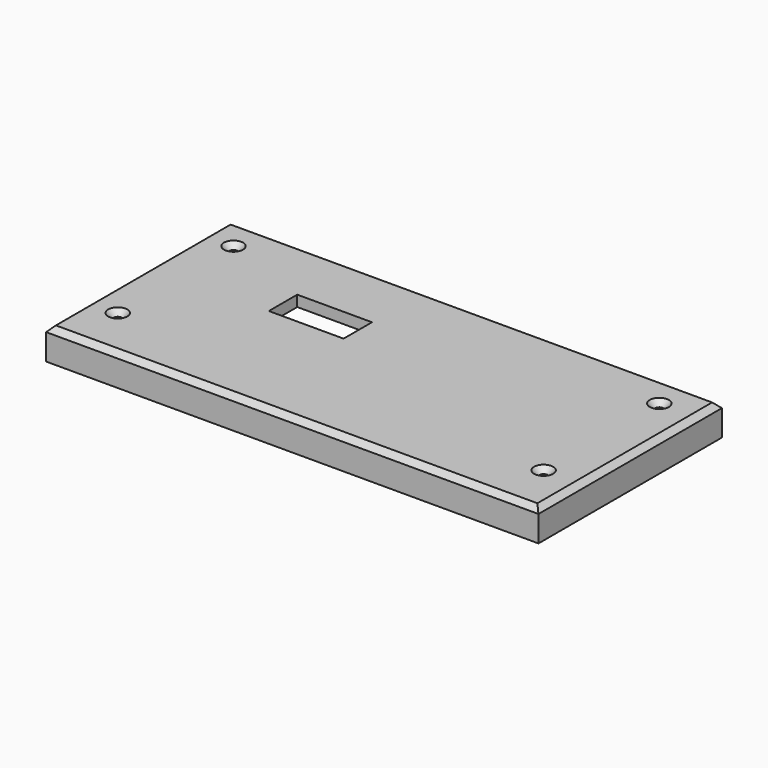
from build123d import *

# Parameters (mm, degrees)
F1_DEPTH = 11.5
F0_R     = 1.5
F2_DEPTH = 4
F3_SIZE  = 2
F4_W     = 27.3790522566
F4_H     = 13
F5_DEPTH = 25


# Not quite as in the source:
# - a feature names something its author has since deleted; it is built from what else it names


with BuildPart() as f1:
    # F0 (on Top) → F1 (new body)
    with BuildSketch(Plane.XY):
        Polygon((-180.3790522566, 0), (0, 0), (0, 42), (0, 84), (-180.3790522566, 84), align=None)
        Polygon((-2, 82), (-2, 42), (-2, 2), (-35, 2), (-178.3790522566, 2), (-178.3790522566, 82), (-35, 82), align=None, mode=Mode.SUBTRACT)
    extrude(amount=-F1_DEPTH)

    # F0 (on Top) → F2 (join)
    with BuildSketch(Plane.XY):
        Polygon((-35, 76.0685783849), (-35, 82), (-178.3790522566, 82), (-178.3790522566, 2), (-35, 2), (-35, 15.0685783849), (-63, 15.0685783849), (-173.3790522566, 15.0685783849), (-173.3790522566, 76.0685783849), align=None)
        with BuildLine():
            Line((-35, 63), (-35, 76.0685783849))
            Line((-35, 76.0685783849), (-173.3790522566, 76.0685783849))
            Line((-173.3790522566, 76.0685783849), (-173.3790522566, 15.0685783849))
            Line((-173.3790522566, 15.0685783849), (-63, 15.0685783849))
            Line((-63, 15.0685783849), (-63, 21.5))
            Line((-63, 21.5), (-163, 21.5))
            Line((-163, 21.5), (-163, 62.5))
            Line((-163, 62.5), (-63, 62.5))
            Line((-63, 62.5), (-63, 42))
            Line((-63, 42), (-56, 42))
            ThreePointArc((-56, 42), (-51, 47), (-46, 42))
            Line((-46, 42), (-40, 42))
            ThreePointArc((-40, 42), (-38.5355339059, 45.5355339059), (-35, 47))
            Line((-35, 47), (-35, 53))
            ThreePointArc((-35, 53), (-40, 58), (-35, 63))
        make_face()
        with Locations((-169.3790522566, 19.0685783849)):
            Circle(F0_R, mode=Mode.SUBTRACT)
        with Locations((-169.3790522566, 72.0685783849)):
            Circle(F0_R, mode=Mode.SUBTRACT)
        with BuildLine():
            Line((-14, 42), (-9.3790522566, 42))
            Line((-9.3790522566, 42), (-9.3790522566, 76.0685783849))
            Line((-9.3790522566, 76.0685783849), (-35, 76.0685783849))
            Line((-35, 76.0685783849), (-35, 63))
            ThreePointArc((-35, 63), (-31.4644660941, 61.5355339059), (-30, 58))
            ThreePointArc((-30, 58), (-31.4644660941, 54.4644660941), (-35, 53))
            Line((-35, 53), (-35, 47))
            ThreePointArc((-35, 47), (-31.4644660941, 45.5355339059), (-30, 42))
            Line((-30, 42), (-24, 42))
            ThreePointArc((-24, 42), (-19, 47), (-14, 42))
        make_face()
        with Locations((-13.3790522566, 72.0685783849)):
            Circle(F0_R, mode=Mode.SUBTRACT)
        Polygon((-9.3790522566, 42), (-2, 42), (-2, 82), (-35, 82), (-35, 76.0685783849), (-9.3790522566, 76.0685783849), align=None)
        Polygon((-2, 2), (-2, 42), (-9.3790522566, 42), (-9.3790522566, 15.0685783849), (-35, 15.0685783849), (-35, 2), align=None)
        with BuildLine():
            Line((-9.3790522566, 15.0685783849), (-9.3790522566, 42))
            Line((-9.3790522566, 42), (-14, 42))
            ThreePointArc((-14, 42), (-19, 37), (-24, 42))
            Line((-24, 42), (-30, 42))
            ThreePointArc((-30, 42), (-31.4644660941, 38.4644660941), (-35, 37))
            Line((-35, 37), (-35, 31))
            ThreePointArc((-35, 31), (-31.4644660941, 29.5355339059), (-30, 26))
            ThreePointArc((-30, 26), (-31.4644660941, 22.4644660941), (-35, 21))
            Line((-35, 21), (-35, 15.0685783849))
            Line((-35, 15.0685783849), (-9.3790522566, 15.0685783849))
        make_face()
        with Locations((-13.3790522566, 19.0685783849)):
            Circle(F0_R, mode=Mode.SUBTRACT)
        with BuildLine():
            Line((-63, 15.0685783849), (-35, 15.0685783849))
            Line((-35, 15.0685783849), (-35, 21))
            ThreePointArc((-35, 21), (-40, 26), (-35, 31))
            Line((-35, 31), (-35, 37))
            ThreePointArc((-35, 37), (-38.5355339059, 38.4644660941), (-40, 42))
            Line((-40, 42), (-46, 42))
            ThreePointArc((-46, 42), (-51, 37), (-56, 42))
            Line((-56, 42), (-63, 42))
            Line((-63, 42), (-63, 21.5))
            Line((-63, 21.5), (-63, 15.0685783849))
        make_face()
        with BuildLine():
            Line((-46, 42), (-56, 42))
            ThreePointArc((-56, 42), (-51, 37), (-46, 42))
        make_face()
        with BuildLine():
            ThreePointArc((-46, 42), (-51, 47), (-56, 42))
            Line((-56, 42), (-46, 42))
        make_face()
        with BuildLine():
            ThreePointArc((-35, 37), (-31.4644660941, 38.4644660941), (-30, 42))
            Line((-30, 42), (-35, 42))
            Line((-35, 42), (-35, 37))
        make_face()
        with BuildLine():
            Line((-35, 42), (-30, 42))
            ThreePointArc((-30, 42), (-31.4644660941, 45.5355339059), (-35, 47))
            Line((-35, 47), (-35, 42))
        make_face()
        with BuildLine():
            ThreePointArc((-40, 42), (-38.5355339059, 38.4644660941), (-35, 37))
            Line((-35, 37), (-35, 42))
            Line((-35, 42), (-40, 42))
        make_face()
        with BuildLine():
            Line((-35, 42), (-35, 47))
            ThreePointArc((-35, 47), (-38.5355339059, 45.5355339059), (-40, 42))
            Line((-40, 42), (-35, 42))
        make_face()
        with BuildLine():
            ThreePointArc((-24, 42), (-19, 37), (-14, 42))
            Line((-14, 42), (-24, 42))
        make_face()
        with BuildLine():
            Line((-24, 42), (-14, 42))
            ThreePointArc((-14, 42), (-19, 47), (-24, 42))
        make_face()
        with BuildLine():
            ThreePointArc((-30, 58), (-31.4644660941, 61.5355339059), (-35, 63))
            Line((-35, 63), (-35, 58))
            Line((-35, 58), (-35, 53))
            ThreePointArc((-35, 53), (-31.4644660941, 54.4644660941), (-30, 58))
        make_face()
        with BuildLine():
            Line((-35, 58), (-35, 63))
            ThreePointArc((-35, 63), (-40, 58), (-35, 53))
            Line((-35, 53), (-35, 58))
        make_face()
        with BuildLine():
            Line((-35, 26), (-35, 21))
            ThreePointArc((-35, 21), (-31.4644660941, 22.4644660941), (-30, 26))
            ThreePointArc((-30, 26), (-31.4644660941, 29.5355339059), (-35, 31))
            Line((-35, 31), (-35, 26))
        make_face()
        with BuildLine():
            ThreePointArc((-35, 31), (-40, 26), (-35, 21))
            Line((-35, 21), (-35, 26))
            Line((-35, 26), (-35, 31))
        make_face()
        Polygon((-163, 21.5), (-63, 21.5), (-63, 42), (-63, 62.5), (-163, 62.5), align=None)
    extrude(amount=-F2_DEPTH)

    # F3
    f3_edges = [f1.edges().sort_by_distance(p)[0] for p in [
        (-90.189526, 84, 0),
        (0, 42, 0),
        (-90.189526, 0, 0),
        (-180.379052, 42, 0),
        (-170.879052, 19.068578, 0),
        (-14.879052, 72.068578, 0),
        (-14.879052, 19.068578, 0),
        (-170.879052, 72.068578, 0),
    ]]
    chamfer(f3_edges, length=F3_SIZE)

    # F4 (on face) → F5 (cut)
    with BuildSketch(Plane.XY):
        with Locations((-122.6895261283, 53.5)):
            Rectangle(F4_W, F4_H)
    extrude(amount=-F5_DEPTH, mode=Mode.SUBTRACT)


solid = f1.part
